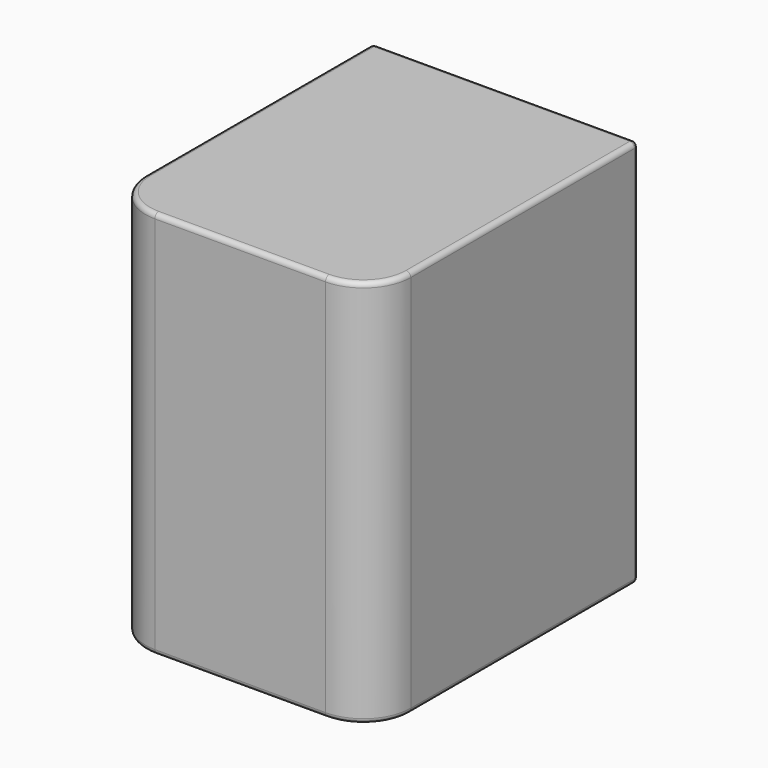
from build123d import *

# Parameters (mm, degrees)
F1_DEPTH = 254
F3_DEPTH = 6.35
F4_F1_R  = 3.175
F4_F2_R  = 3.1749


# Not quite as in the source:
# - a fillet or chamfer is up to 0.001 mm smaller than in the source, because OpenCascade refuses the exact size


with BuildPart() as f1:
    # F0 (on Top) → F1 (new body)
    with BuildSketch(Plane.XY):
        with BuildLine():
            Line((57.15, -215.9), (-57.15, -215.9))
            ThreePointArc((-57.15, -215.9), (-75.1105122421, -208.4605122421), (-82.55, -190.5))
            Line((-82.55, -190.5), (-82.55, 0))
            Line((-82.55, 0), (-88.9, 0))
            Line((-88.9, 0), (-88.9, -190.5))
            ThreePointArc((-88.9, -190.5), (-79.6006403027, -212.9506403027), (-57.15, -222.25))
            Line((-57.15, -222.25), (57.15, -222.25))
            ThreePointArc((57.15, -222.25), (79.6006403027, -212.9506403027), (88.9, -190.5))
            Line((88.9, -190.5), (88.9, 0))
            Line((88.9, 0), (82.55, 0))
            Line((82.55, 0), (82.55, -190.5))
            ThreePointArc((82.55, -190.5), (75.1105122421, -208.4605122421), (57.15, -215.9))
        make_face()
    extrude(amount=F1_DEPTH)

    # F2 (on face) → F3 (join)
    with BuildSketch(Plane.XY.offset(254)):
        with BuildLine():
            Line((82.55, 0), (-82.55, 0))
            Line((-82.55, 0), (-82.55, -190.5))
            ThreePointArc((-82.55, -190.5), (-75.1105122421, -208.4605122421), (-57.15, -215.9))
            Line((-57.15, -215.9), (57.15, -215.9))
            ThreePointArc((57.15, -215.9), (75.1105122421, -208.4605122421), (82.55, -190.5))
            Line((82.55, -190.5), (82.55, 0))
        make_face()
        with BuildLine():
            Line((-82.55, 0), (-88.9, 0))
            Line((-88.9, 0), (-88.9, -190.5))
            ThreePointArc((-88.9, -190.5), (-79.6006403027, -212.9506403027), (-57.15, -222.25))
            Line((-57.15, -222.25), (57.15, -222.25))
            ThreePointArc((57.15, -222.25), (79.6006403027, -212.9506403027), (88.9, -190.5))
            Line((88.9, -190.5), (88.9, 0))
            Line((88.9, 0), (82.55, 0))
            Line((82.55, 0), (82.55, -190.5))
            ThreePointArc((82.55, -190.5), (75.1105122421, -208.4605122421), (57.15, -215.9))
            Line((57.15, -215.9), (-57.15, -215.9))
            ThreePointArc((-57.15, -215.9), (-75.1105122421, -208.4605122421), (-82.55, -190.5))
            Line((-82.55, -190.5), (-82.55, 0))
        make_face()
    extrude(amount=F3_DEPTH)

    # F4: fillet of radius 3.175 on 23 edges, made by hand

    # F4_f1
    f4_f1_edges = [f1.edges().sort_by_distance(p)[0] for p in [
        (75.1105122421, -208.4605122421, 254),
        (82.55, -95.25, 254),
        (0, -215.9, 254),
        (-75.1105122421, -208.4605122421, 254),
        (-82.55, -95.25, 254),
    ]]
    fillet(f4_f1_edges, radius=F4_F1_R)

    # F4_f2 (radius 3.175 in the source; OpenCascade refuses exactly that, so slightly less here)
    f4_f2_edges = [f1.edges().sort_by_distance(p)[0] for p in [
        (-88.9, -95.25, 260.35),
        (-79.6006403027, -212.9506403027, 260.35),
        (0, -222.25, 260.35),
        (79.6006403027, -212.9506403027, 260.35),
        (88.9, -95.25, 260.35),
        (0, 0, 260.35),
        (88.9, 0, 130.175),
        (-88.9, 0, 130.175),
        (82.55, 0, 125.4125),
        (-82.55, 0, 125.4125),
        (75.1105122421, -208.4605122421, 0),
        (0, -215.9, 0),
        (-75.1105122421, -208.4605122421, 0),
        (-82.55, -95.25, 0),
        (-85.725, 0, 0),
        (-88.9, -95.25, 0),
        (-79.6006403027, -212.9506403027, 0),
        (0, -222.25, 0),
        (79.6006403027, -212.9506403027, 0),
        (88.9, -95.25, 0),
        (85.725, 0, 0),
        (82.55, -95.25, 0),
        (-81.6200640303, 0, 253.0700640303),
        (81.6200640303, 0, 253.0700640303),
    ]]
    fillet(f4_f2_edges, radius=F4_F2_R)


solid = f1.part
